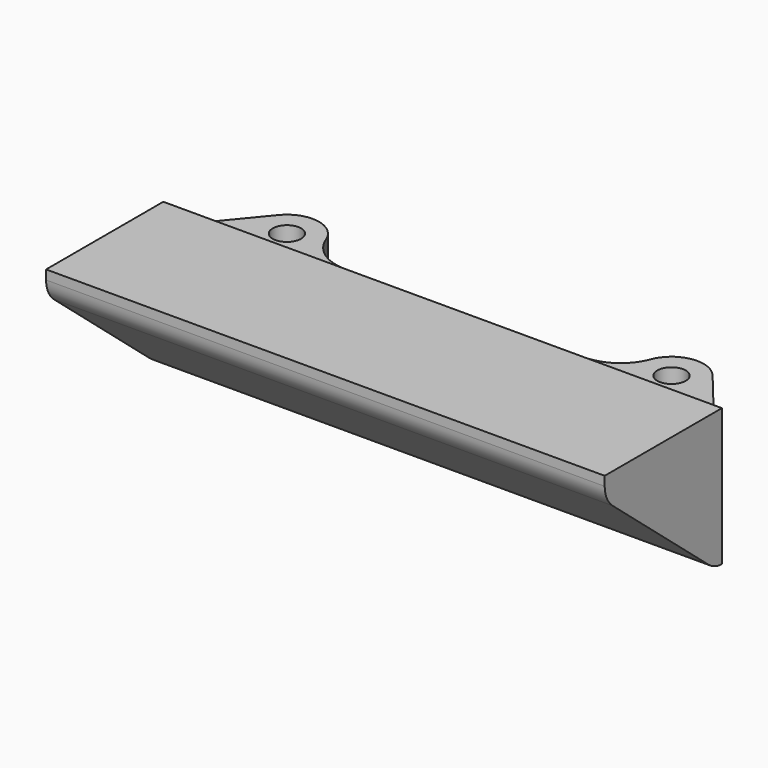
from build123d import *

# Parameters (mm, degrees)
F1_DEPTH    = 7.5
F2_DEPTH    = 5.5
F3_SIZE2    = 12.5864944677
F3_SIZE     = 15
F5_D        = 3.1
F6_R        = 3
F7_T1_DEPTH = 66.4481797844
F7_T3_DEPTH = 16.376963756
F8_R        = 5


# Not quite as in the source:
# - a fillet or chamfer that OpenCascade refuses, or shapes differently, is made with other operations: its cross-section is extruded or revolved along the edge and cut away or added


with BuildPart() as f1:
    # F0 (on Top) → F1 (new body, symmetric)
    with BuildSketch(Plane.XY):
        Polygon((28, 0), (0, 0), (0, -16), (30.5, -16), (30.5, 0), align=None)
        Polygon((0, 0), (-28, 0), (-30.5, 0), (-30.5, -16), (0, -16), align=None)
    extrude(amount=F1_DEPTH, both=True)

    # F0 (on Top) → F2 (join, symmetric)
    with BuildSketch(Plane.XY):
        with BuildLine():
            Line((-17.5, 3), (-17.5, 5))
            ThreePointArc((-17.5, 5), (-22.1810377062, 1.7052845439), (-23.7029428208, 7.2235332486))
            Line((-23.7029428208, 7.2235332486), (-28, 2))
            Line((-28, 2), (-28, 0))
            Line((-28, 0), (0, 0))
            Line((0, 0), (0, 3))
            Line((0, 3), (-17.5, 3))
        make_face()
        with BuildLine():
            ThreePointArc((-23.7029428208, 7.2235332486), (-22.1810377062, 1.7052845439), (-17.5, 5))
            ThreePointArc((-17.5, 5), (-19.8189622938, 8.2947154561), (-23.7029428208, 7.2235332486))
        make_face()
        with BuildLine():
            ThreePointArc((23.7029428208, 7.2235332486), (19.8189622938, 8.2947154561), (17.5, 5))
            ThreePointArc((17.5, 5), (21, 1.5), (24.5, 5))
            ThreePointArc((24.5, 5), (24.2947154561, 6.1810377062), (23.7029428208, 7.2235332486))
        make_face()
        with BuildLine():
            Line((17.5, 3), (0, 3))
            Line((0, 3), (0, 0))
            Line((0, 0), (28, 0))
            Line((28, 0), (28, 2))
            Line((28, 2), (23.7029428208, 7.2235332486))
            ThreePointArc((23.7029428208, 7.2235332486), (24.2947154561, 6.1810377062), (24.5, 5))
            ThreePointArc((24.5, 5), (21, 1.5), (17.5, 5))
            Line((17.5, 5), (17.5, 3))
        make_face()
    extrude(amount=F2_DEPTH, both=True)

    # F3
    f3_edges = [f1.edges().sort_by_distance(p)[0] for p in [
        (0, -16, -7.5),
    ]]
    f3_side = f1.faces().sort_by_distance((0, -8, -7.5))[0]
    chamfer(f3_edges, length=F3_SIZE, length2=F3_SIZE2, reference=f3_side)

    # F5 (through all)
    with Locations(Plane.XY.offset(5.5)):
        with Locations((-21, 5), (21, 5)):
            Hole(F5_D / 2)

    # F6
    f6_edges = [f1.edges().sort_by_distance(p)[0] for p in [
        (0, -16, 5.086494),
    ]]
    fillet(f6_edges, radius=F6_R)

    # F7: fillet of radius 3 on 3 edges, made by hand

    # F7_s2 → F7_t1 (cut)
    with BuildSketch(Plane.YZ.offset(-33.2240898922)):
        with BuildLine():
            ThreePointArc((-1.8347095698, -6.7995955078), (-0.9762901404, -7.3041789179), (0, -7.5))
            Line((0, -7.5), (-1, -7.5))
            Line((-1, -7.5), (-1.8347095698, -6.7995955078))
        make_face()
    extrude(amount=F7_T1_DEPTH, mode=Mode.SUBTRACT)

    # F7_s4 → F7_t3 (cut)
    with BuildSketch(Plane.XY.offset(-8.188481878)):
        with BuildLine():
            ThreePointArc((-28, 0.9246072488), (-27.8240418195, 1.9369252827), (-27.3168081321, 2.8304928904))
            Line((-27.3168081321, 2.8304928904), (-28, 2))
            Line((-28, 2), (-28, 0.9246072488))
        make_face()
        with BuildLine():
            ThreePointArc((28, 0.9246072488), (27.8240418195, 1.9369252827), (27.3168081321, 2.8304928904))
            Line((27.3168081321, 2.8304928904), (28, 2))
            Line((28, 2), (28, 0.9246072488))
        make_face()
    extrude(amount=F7_T3_DEPTH, mode=Mode.SUBTRACT)

    # F8
    f8_edges = [f1.edges().sort_by_distance(p)[0] for p in [
        (17.5, 3, 0),
        (-17.5, 3, 0),
    ]]
    fillet(f8_edges, radius=F8_R)


solid = f1.part
